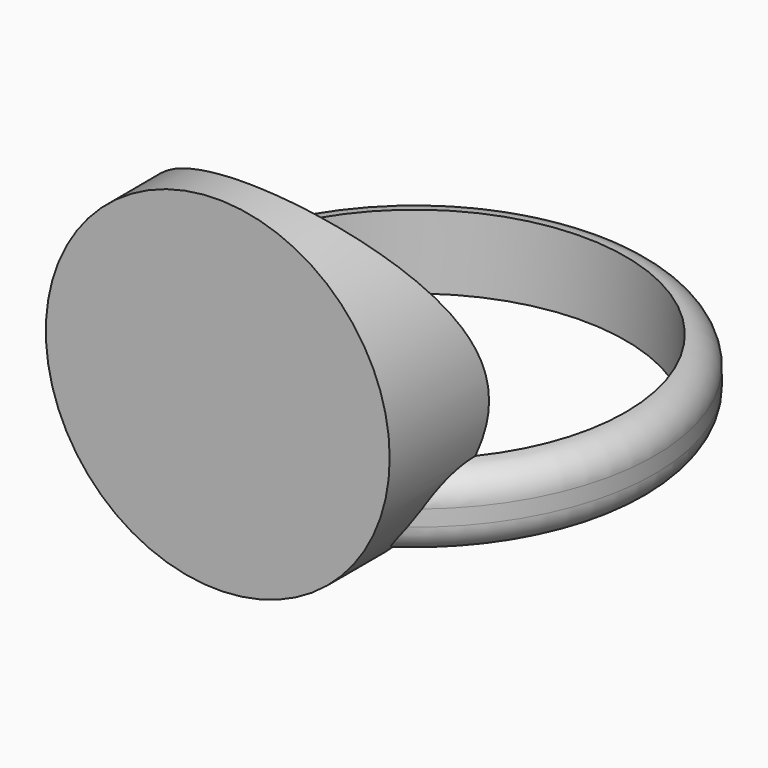
from build123d import *

# Parameters (mm, degrees)
F0_R     = 42.0549170166
F1_DEPTH = 12.954
F2_R     = 5.08
F4_R     = 30.1481321403
F5_DEPTH = 43.18
F6_R     = 36.9749170166
F7_DEPTH = 77.47
F8_R     = 36.9749170166
F9_DEPTH = 29.464


# Not quite as in the source:
# - a feature of the source that left no trace in its solid (it failed there, or was rolled back) is left out


with BuildPart() as f1:
    # F0 (on Top) → F1 (new body)
    with BuildSketch(Plane.XY):
        Circle(F0_R)
    extrude(amount=F1_DEPTH)

    # F2
    f2_edges = [f1.edges().sort_by_distance(p)[0] for p in [
        (-42.054917, 0, 12.954),
        (-42.054917, 0, 0),
    ]]
    fillet(f2_edges, radius=F2_R)

    # F4 (on Front) → F5 (join)
    with BuildSketch(Plane.XZ):
        with Locations((0, 21.2246719748)):
            Circle(F4_R)
    extrude(amount=F5_DEPTH)

    # F6 (on Top) → F7 (cut)
    with BuildSketch(Plane.XY):
        Circle(F6_R)
    extrude(amount=F7_DEPTH, mode=Mode.SUBTRACT)

    # F8 (on Top) → F9 (cut)
    with BuildSketch(Plane.XY):
        Circle(F8_R)
    extrude(amount=-F9_DEPTH, mode=Mode.SUBTRACT)


solid = f1.part
